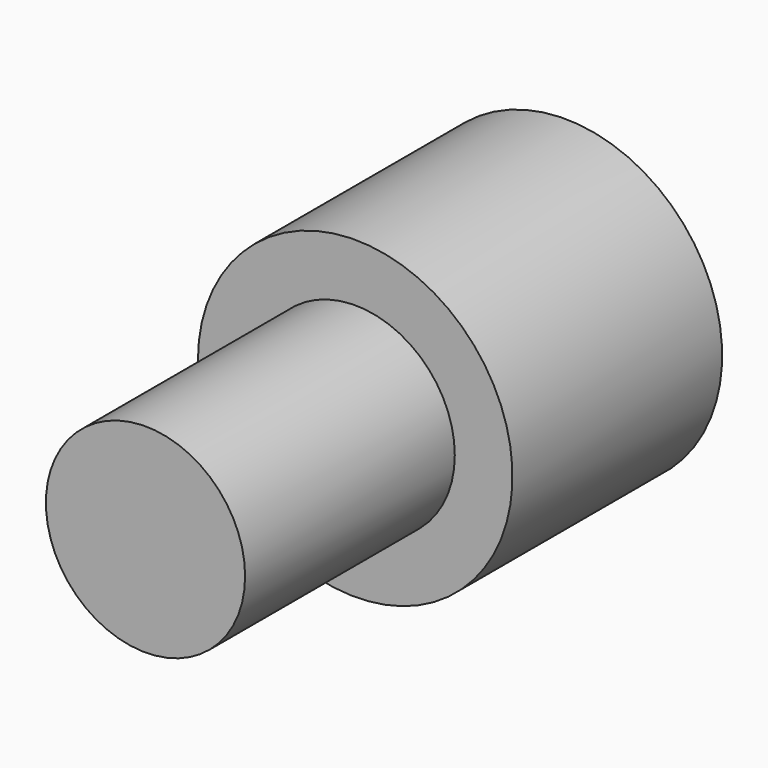
from build123d import *

# Parameters (mm, degrees)
F0_R     = 9.5
F1_DEPTH = 25
F2_R     = 15
F2_R_2   = 9.5
F3_DEPTH = 25


with BuildPart() as f1:
    # F0 (on Front) → F1 (new body)
    with BuildSketch(Plane.XZ):
        Circle(F0_R)
    extrude(amount=-F1_DEPTH)

    # F2 (on face) → F3 (join)
    with BuildSketch(Plane(origin=(0, 25, 0), x_dir=(-1, 0, 0), z_dir=(0, 1, 0))):
        Circle(F2_R)
        Circle(F2_R_2, mode=Mode.SUBTRACT)
        Circle(F2_R_2)
    extrude(amount=F3_DEPTH)


solid = f1.part
